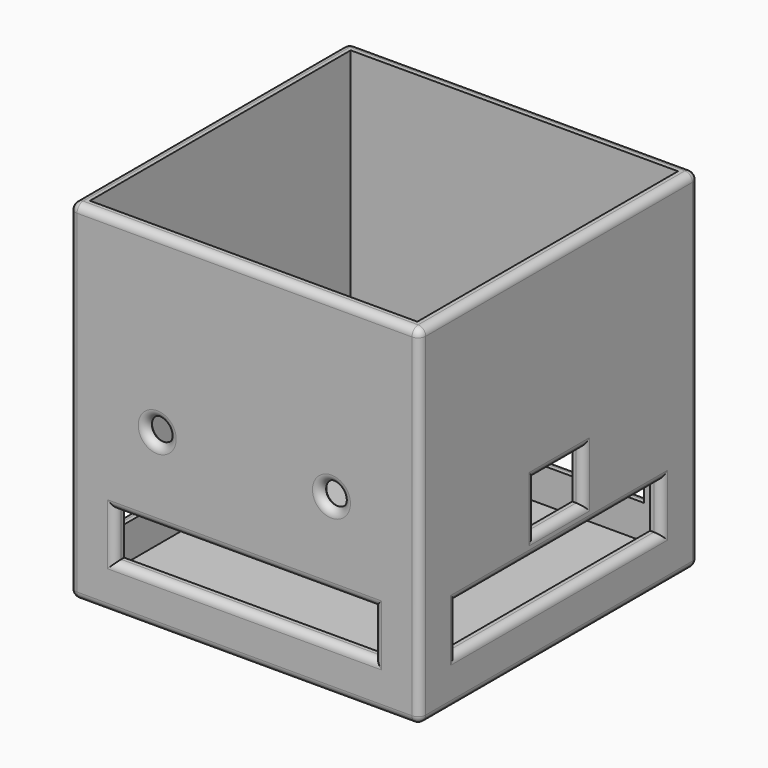
from build123d import *

# Parameters (mm, degrees)
F0_W      = 4.61
F0_H      = 4.59
F1_DEPTH  = 4.59
F2_T      = -0.15
F3_R      = 0.15
F4_DEPTH  = 0.2
F5_W      = 3.41
F5_H      = 0.6
F6_DEPTH  = 4.7
F7_W      = 3.3708
F7_H      = 0.6096
F8_DEPTH  = 4.7
F9_W      = 0.8
F9_H      = 0.65
F10_DEPTH = 4.7
F11_R     = 0.1


# Not quite as in the source:
# - a fillet or chamfer that OpenCascade refuses, or shapes differently, is made with other operations: its cross-section is extruded or revolved along the edge and cut away or added


with BuildPart() as f1:
    # F0 (on Front) → F1 (new body)
    with BuildSketch(Plane.XZ):
        Rectangle(F0_W, F0_H)
    extrude(amount=F1_DEPTH)

    # F2
    f2_openings = [f1.faces().sort_by_distance(p)[0] for p in [
        (0, -2.295, 2.295),
    ]]
    offset(amount=F2_T, openings=f2_openings)

    # F3 (on face) → F4 (cut)
    with BuildSketch(Plane.XZ.offset(4.59)):
        with Locations((1.1442566571, 0)):
            Circle(F3_R)
        with Locations((-1.1498022541, 0)):
            Circle(F3_R)
    extrude(amount=-F4_DEPTH, mode=Mode.SUBTRACT)

    # F5 (on face) → F6 (cut)
    with BuildSketch(Plane(origin=(0, 0, 0), x_dir=(-1, 0, 0), z_dir=(0, 1, 0))):
        with Locations((0, -1.395)):
            Rectangle(F5_W, F5_H)
    extrude(amount=-F6_DEPTH, mode=Mode.SUBTRACT)

    # F7 (on face) → F8 (cut)
    with BuildSketch(Plane(origin=(-2.305, 0, 0), x_dir=(0, -1, 0), z_dir=(-1, 0, 0))):
        with Locations((2.295, -1.3806)):
            Rectangle(F7_W, F7_H)
    extrude(amount=-F8_DEPTH, mode=Mode.SUBTRACT)

    # F9 (on face) → F10 (cut)
    with BuildSketch(Plane.YZ.offset(2.305)):
        with Locations((-2.29, -0.5008)):
            Rectangle(F9_W, F9_H)
    extrude(amount=-F10_DEPTH, mode=Mode.SUBTRACT)

    # F11
    f11_edges = [f1.edges().sort_by_distance(p)[0] for p in [
        (0, -4.59, 2.295),
        (2.305, -4.59, 0),
        (-2.305, -4.59, 0),
        (0, -4.59, -2.295),
        (0, -4.59, -1.095),
        (-1.705, -4.59, -1.395),
        (0, -4.59, -1.695),
        (1.705, -4.59, -1.395),
        (-1.299802, -4.59, 0),
        (0.994257, -4.59, 0),
        (2.305, -2.295, -2.295),
        (2.305, 0, 0),
        (2.305, -2.295, 2.295),
        (2.305, -2.295, -1.0758),
        (2.305, -3.9804, -1.3806),
        (2.305, -0.6096, -1.3806),
        (2.305, -2.295, -1.6854),
        (2.305, -2.29, -0.8258),
        (2.305, -2.69, -0.5008),
        (2.305, -2.29, -0.1758),
        (2.305, -1.89, -0.5008),
        (0, 0, 2.295),
        (-2.305, 0, 0),
        (0, 0, -2.295),
        (-1.705, 0, -1.395),
        (0, 0, -1.695),
        (1.705, 0, -1.395),
        (0, 0, -1.095),
        (-2.305, -2.295, 2.295),
        (-2.305, -2.295, -2.295),
        (-2.305, -3.9804, -1.3806),
        (-2.305, -2.295, -1.6854),
        (-2.305, -2.295, -1.0758),
        (-2.305, -0.6096, -1.3806),
        (-2.305, -1.89, -0.5008),
        (-2.305, -2.29, -0.1758),
        (-2.305, -2.69, -0.5008),
        (-2.305, -2.29, -0.8258),
    ]]
    fillet(f11_edges, radius=F11_R)

    # F12: fillet of radius 0.1 on 2 edges, made by hand

    # F12_s1 → F12_t2 (revolve, cut)
    with BuildSketch(Plane.XY):
        with BuildLine():
            ThreePointArc((1.3808591975, -4.44), (1.3308591975, -4.4533974596), (1.2942566571, -4.49))
            Line((1.2942566571, -4.49), (1.2942566571, -4.44))
            Line((1.2942566571, -4.44), (1.3808591975, -4.44))
        make_face()
    revolve(axis=Axis((1.1442566571, -4.44, 0), (0, -1, 0)), mode=Mode.SUBTRACT)

    # F12_s3 → F12_t4 (revolve, cut)
    with BuildSketch(Plane.XY):
        with BuildLine():
            ThreePointArc((-0.9131997137, -4.44), (-0.9631997137, -4.4533974596), (-0.9998022541, -4.49))
            Line((-0.9998022541, -4.49), (-0.9998022541, -4.44))
            Line((-0.9998022541, -4.44), (-0.9131997137, -4.44))
        make_face()
    revolve(axis=Axis((-1.1498022541, -4.44, 0), (0, -1, 0)), mode=Mode.SUBTRACT)


solid = f1.part
